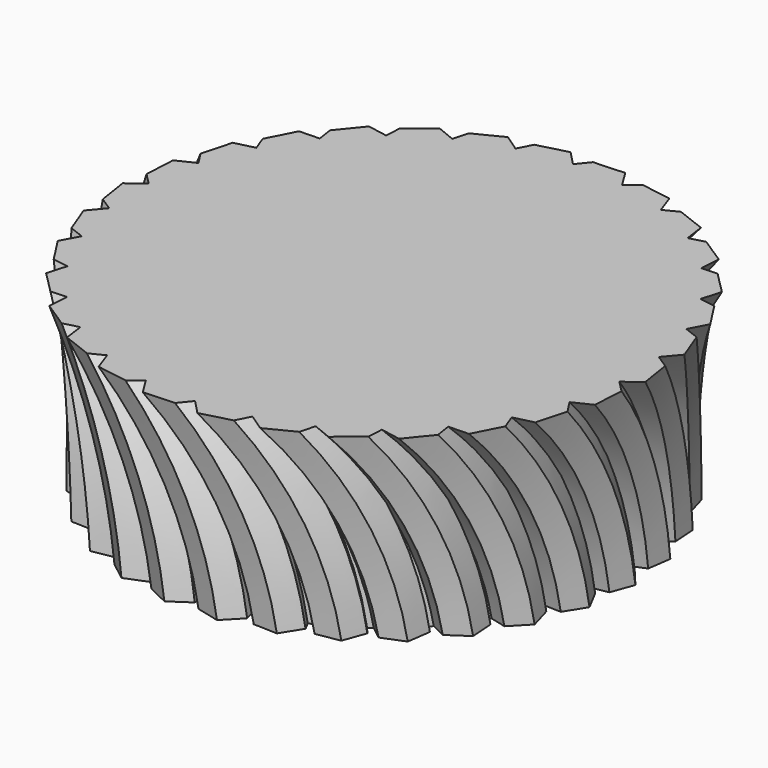
from build123d import *

# Parameters (mm, degrees)
F5_COUNT = 30
F6_R     = 30
F7_DEPTH = 25
F8_R     = 86.1433169454
F9_DEPTH = 25


with BuildPart() as f4:
    # F4: sweep along a path in F2
    with BuildLine(Plane.YZ.offset(-30)) as f4_path:
        ThreePointArc((13.1748821586, 26.7821643502), (4.4397694253, 14.4475808429), (0, 0))
    # F0 (on Top) → F4 (sweep)
    with BuildSketch(Plane.XY):
        Polygon((-32.0411247972, 2.43251781), (-33.1271846172, -0.5514070217), (-31.08605982, -2.9839248316), (-27.9588752028, -2.43251781), (-26.8728153828, 0.5514070217), (-28.91394018, 2.9839248316), align=None)
        Polygon((-17.6281463431, 1.8192284857), (-28.91394018, 2.9839248316), (-26.8728153828, 0.5514070217), (-27.9588752028, -2.43251781), (-17.6281463431, -1.5337090503), align=None)
    sweep(path=f4_path.line)

    # F5: F4 ×30 about axis
    f5_axis = Axis((0, 0, 15.9086212516), (0, 0, 1))


with BuildPart() as f4_1:
    add(f4.part)
    for i in range(1, F5_COUNT):
        add(f4.part.rotate(f5_axis, i * 360 / F5_COUNT))

    # F6 (on Top) → F7 (join)
    with BuildSketch(Plane.XY):
        Circle(F6_R)
    extrude(amount=F7_DEPTH)

    # F8 (on face) → F9 (cut)
    with BuildSketch(Plane.XY.offset(25)):
        Circle(F8_R)
        with BuildLine():
            Line((-17.6281463431, 9.5111030199), (-17.6281463431, 13.1997105208))
            add(Edge.make_bspline(
                [(-17.6281463436, 13.1997105151), (-17.03748869, 13.1417822064), (-16.4468217334, 13.0839139825), (-15.8561453818, 13.0261064694), (-15.2654595405, 12.9683603114)],
                knots=[0.771630404, 0.771630404, 0.771630404, 0.771630404, 0.771630404, 1, 1, 1, 1, 1], degree=4))
            Line((-15.2654595405, 12.9683603114), (-14.4985549182, 16.5763628885))
            add(Edge.make_bspline(
                [(-14.4985549199, 16.5763628831), (-13.9328485257, 16.3968958154), (-13.3671205396, 16.2174855854), (-12.8013707413, 16.0381327862), (-12.2355989041, 15.8588380282)],
                knots=[0.771630404, 0.771630404, 0.771630404, 0.771630404, 0.771630404, 1, 1, 1, 1, 1], degree=4))
            Line((-12.2355989041, 15.8588380282), (-10.7353070716, 19.2285486557))
            add(Edge.make_bspline(
                [(-10.7353070744, 19.2285486508), (-10.2192760237, 18.9353863962), (-9.7032120357, 18.642275248), (-9.1871147716, 18.3492157407), (-8.6709838828, 18.0562084241)],
                knots=[0.771630404, 0.771630404, 0.771630404, 0.771630404, 0.771630404, 1, 1, 1, 1, 1], degree=4))
            Line((-8.6709838828, 18.0562084241), (-6.5028747922, 21.0403545779))
            add(Edge.make_bspline(
                [(-6.502874796, 21.0403545736), (-6.0590721219, 20.6463097294), (-5.6152266046, 20.2523080268), (-5.1713378016, 19.858349918), (-4.7274052577, 19.4644358685)],
                knots=[0.771630404, 0.771630404, 0.771630404, 0.771630404, 0.771630404, 1, 1, 1, 1, 1], degree=4))
            Line((-4.7274052577, 19.4644358685), (-1.9862356802, 21.9325960422))
            add(Edge.make_bspline(
                [(-1.9862356848, 21.9325960388), (-1.6340576937, 21.4548902555), (-1.2818288261, 20.9772177634), (-0.929548555, 20.4995789129), (-0.5772163383, 20.0219740647)],
                knots=[0.771630404, 0.771630404, 0.771630404, 0.771630404, 0.771630404, 1, 1, 1, 1, 1], degree=4))
            Line((-0.5772163383, 20.0219740647), (2.617211462, 21.8662778151))
            add(Edge.make_bspline(
                [(2.6172114569, 21.8662778128), (2.8623728968, 21.3257891254), (3.1075910231, 20.7853224239), (3.352866424, 20.2448779415), (3.5981997049, 19.7044559182)],
                knots=[0.771630404, 0.771630404, 0.771630404, 0.771630404, 0.771630404, 1, 1, 1, 1, 1], degree=4))
            Line((3.5981997049, 19.7044559182), (7.1062739047, 20.8442983215))
            add(Edge.make_bspline(
                [(7.1062738991, 20.8442983203), (7.2337040565, 20.264648678), (7.3611942326, 19.6850087554), (7.4887450515, 19.1053786583), (7.6163571549, 18.5257584956)],
                knots=[0.771630404, 0.771630404, 0.771630404, 0.771630404, 0.771630404, 1, 1, 1, 1, 1], degree=4))
            Line((7.6163571549, 18.5257584956), (11.2847580779, 18.9113229693))
            add(Edge.make_bspline(
                [(11.2847580723, 18.9113229692), (11.2888876377, 18.3178458429), (11.2930779313, 17.7243657452), (11.2973295851, 17.13088265), (11.3016432499, 16.5373965303)],
                knots=[0.771630404, 0.771630404, 0.771630404, 0.771630404, 0.771630404, 1, 1, 1, 1, 1], degree=4))
            Line((11.3016432499, 16.5373965303), (14.9700441729, 16.1518320566))
            add(Edge.make_bspline(
                [(14.9700441674, 16.1518320578), (14.8506926591, 15.5704652456), (14.7313999341, 14.989082901), (14.6121666054, 14.4076848668), (14.4929933036, 13.8262709814)],
                knots=[0.771630404, 0.771630404, 0.771630404, 0.771630404, 0.771630404, 1, 1, 1, 1, 1], degree=4))
            Line((14.4929933036, 13.8262709814), (18.0010675033, 12.686428578))
            add(Edge.make_bspline(
                [(18.0010674981, 12.6864285803), (17.7634511498, 12.1425806017), (17.5258890708, 11.5987052084), (17.288381828, 11.0548021191), (17.0509300048, 10.5108710448)],
                knots=[0.771630404, 0.771630404, 0.771630404, 0.771630404, 0.771630404, 1, 1, 1, 1, 1], degree=4))
            Line((17.0509300048, 10.5108710448), (20.2453578051, 8.6665672944))
            add(Edge.make_bspline(
                [(20.2453578005, 8.6665672977), (19.8998615867, 8.184006919), (19.5544127565, 7.7014084414), (19.2090118059, 7.218771472), (18.8636592453, 6.7360956068)],
                knots=[0.771630404, 0.771630404, 0.771630404, 0.771630404, 0.771630404, 1, 1, 1, 1, 1], degree=4))
            Line((18.8636592453, 6.7360956068), (21.6048288228, 4.2679354331))
            add(Edge.make_bspline(
                [(21.604828819, 4.2679354373), (21.1665525822, 3.8677528627), (20.7283147722, 3.4675231701), (20.2901157927, 3.0672458721), (19.851956059, 2.6669204674)],
                knots=[0.771630404, 0.771630404, 0.771630404, 0.771630404, 0.771630404, 1, 1, 1, 1, 1], degree=4))
            Line((19.851956059, 2.6669204674), (22.0200651495, -0.3172256864))
            add(Edge.make_bspline(
                [(22.0200651467, -0.3172256815), (21.5081636614, -0.6175405533), (20.996289967, -0.9179095028), (20.4844443567, -1.2183330907), (19.9726271326, -1.5188118938)],
                knots=[0.771630404, 0.771630404, 0.771630404, 0.771630404, 0.771630404, 1, 1, 1, 1, 1], degree=4))
            Line((19.9726271326, -1.5188118938), (21.4729189652, -4.8885225212))
            add(Edge.make_bspline(
                [(21.4729189634, -4.8885225158), (20.909764781, -5.0758444838), (20.3466265388, -5.2632251258), (19.783504407, -5.4506650512), (19.2203985613, -5.6381648871)],
                knots=[0.771630404, 0.771630404, 0.771630404, 0.771630404, 0.771630404, 1, 1, 1, 1, 1], degree=4))
            Line((19.2203985613, -5.6381648871), (19.9873031836, -9.2461674641))
            add(Edge.make_bspline(
                [(19.9873031829, -9.2461674585), (19.3975088435, -9.3123096537), (18.8077178969, -9.378512555), (18.217930383, -9.4447767938), (17.6281463431, -9.5111030199)],
                knots=[0.771630404, 0.771630404, 0.771630404, 0.771630404, 0.771630404, 1, 1, 1, 1, 1], degree=4))
            Line((17.6281463431, -9.5111030199), (17.6281463431, -13.1997105208))
            add(Edge.make_bspline(
                [(17.6281463436, -13.1997105151), (17.03748869, -13.1417822064), (16.4468217334, -13.0839139825), (15.8561453818, -13.0261064694), (15.2654595405, -12.9683603114)],
                knots=[0.771630404, 0.771630404, 0.771630404, 0.771630404, 0.771630404, 1, 1, 1, 1, 1], degree=4))
            Line((15.2654595405, -12.9683603114), (14.4985549182, -16.5763628885))
            add(Edge.make_bspline(
                [(14.4985549199, -16.5763628831), (13.9328485257, -16.3968958154), (13.3671205396, -16.2174855854), (12.8013707413, -16.0381327862), (12.2355989041, -15.8588380282)],
                knots=[0.771630404, 0.771630404, 0.771630404, 0.771630404, 0.771630404, 1, 1, 1, 1, 1], degree=4))
            Line((12.2355989041, -15.8588380282), (10.7353070716, -19.2285486557))
            add(Edge.make_bspline(
                [(10.7353070744, -19.2285486508), (10.2192760237, -18.9353863962), (9.7032120357, -18.642275248), (9.1871147716, -18.3492157407), (8.6709838828, -18.0562084241)],
                knots=[0.771630404, 0.771630404, 0.771630404, 0.771630404, 0.771630404, 1, 1, 1, 1, 1], degree=4))
            Line((8.6709838828, -18.0562084241), (6.5028747922, -21.0403545779))
            add(Edge.make_bspline(
                [(6.502874796, -21.0403545736), (6.0590721219, -20.6463097294), (5.6152266046, -20.2523080268), (5.1713378016, -19.858349918), (4.7274052577, -19.4644358685)],
                knots=[0.771630404, 0.771630404, 0.771630404, 0.771630404, 0.771630404, 1, 1, 1, 1, 1], degree=4))
            Line((4.7274052577, -19.4644358685), (1.9862356802, -21.9325960422))
            add(Edge.make_bspline(
                [(1.9862356848, -21.9325960388), (1.6340576937, -21.4548902555), (1.2818288261, -20.9772177634), (0.929548555, -20.4995789129), (0.5772163383, -20.0219740647)],
                knots=[0.771630404, 0.771630404, 0.771630404, 0.771630404, 0.771630404, 1, 1, 1, 1, 1], degree=4))
            Line((0.5772163383, -20.0219740647), (-2.617211462, -21.8662778151))
            add(Edge.make_bspline(
                [(-2.6172114569, -21.8662778128), (-2.8623728968, -21.3257891254), (-3.1075910231, -20.7853224239), (-3.352866424, -20.2448779415), (-3.5981997049, -19.7044559182)],
                knots=[0.771630404, 0.771630404, 0.771630404, 0.771630404, 0.771630404, 1, 1, 1, 1, 1], degree=4))
            Line((-3.5981997049, -19.7044559182), (-7.1062739047, -20.8442983215))
            add(Edge.make_bspline(
                [(-7.1062738991, -20.8442983203), (-7.2337040565, -20.264648678), (-7.3611942326, -19.6850087554), (-7.4887450515, -19.1053786583), (-7.6163571549, -18.5257584956)],
                knots=[0.771630404, 0.771630404, 0.771630404, 0.771630404, 0.771630404, 1, 1, 1, 1, 1], degree=4))
            Line((-7.6163571549, -18.5257584956), (-11.2847580779, -18.9113229693))
            add(Edge.make_bspline(
                [(-11.2847580723, -18.9113229692), (-11.2888876377, -18.3178458429), (-11.2930779313, -17.7243657452), (-11.2973295851, -17.13088265), (-11.3016432499, -16.5373965303)],
                knots=[0.771630404, 0.771630404, 0.771630404, 0.771630404, 0.771630404, 1, 1, 1, 1, 1], degree=4))
            Line((-11.3016432499, -16.5373965303), (-14.9700441729, -16.1518320566))
            add(Edge.make_bspline(
                [(-14.9700441674, -16.1518320578), (-14.8506926591, -15.5704652456), (-14.7313999341, -14.989082901), (-14.6121666054, -14.4076848668), (-14.4929933036, -13.8262709814)],
                knots=[0.771630404, 0.771630404, 0.771630404, 0.771630404, 0.771630404, 1, 1, 1, 1, 1], degree=4))
            Line((-14.4929933036, -13.8262709814), (-18.0010675033, -12.686428578))
            add(Edge.make_bspline(
                [(-18.0010674981, -12.6864285803), (-17.7634511498, -12.1425806017), (-17.5258890708, -11.5987052084), (-17.288381828, -11.0548021191), (-17.0509300048, -10.5108710448)],
                knots=[0.771630404, 0.771630404, 0.771630404, 0.771630404, 0.771630404, 1, 1, 1, 1, 1], degree=4))
            Line((-17.0509300048, -10.5108710448), (-20.2453578051, -8.6665672944))
            add(Edge.make_bspline(
                [(-20.2453578005, -8.6665672977), (-19.8998615867, -8.184006919), (-19.5544127565, -7.7014084414), (-19.2090118059, -7.218771472), (-18.8636592453, -6.7360956068)],
                knots=[0.771630404, 0.771630404, 0.771630404, 0.771630404, 0.771630404, 1, 1, 1, 1, 1], degree=4))
            Line((-18.8636592453, -6.7360956068), (-21.6048288228, -4.2679354331))
            add(Edge.make_bspline(
                [(-21.604828819, -4.2679354373), (-21.1665525822, -3.8677528627), (-20.7283147722, -3.4675231701), (-20.2901157927, -3.0672458721), (-19.851956059, -2.6669204674)],
                knots=[0.771630404, 0.771630404, 0.771630404, 0.771630404, 0.771630404, 1, 1, 1, 1, 1], degree=4))
            Line((-19.851956059, -2.6669204674), (-22.0200651495, 0.3172256864))
            add(Edge.make_bspline(
                [(-22.0200651467, 0.3172256815), (-21.5081636614, 0.6175405533), (-20.996289967, 0.9179095028), (-20.4844443567, 1.2183330907), (-19.9726271326, 1.5188118938)],
                knots=[0.771630404, 0.771630404, 0.771630404, 0.771630404, 0.771630404, 1, 1, 1, 1, 1], degree=4))
            Line((-19.9726271326, 1.5188118938), (-21.4729189652, 4.8885225212))
            add(Edge.make_bspline(
                [(-21.4729189634, 4.8885225158), (-20.909764781, 5.0758444838), (-20.3466265388, 5.2632251258), (-19.783504407, 5.4506650512), (-19.2203985613, 5.6381648871)],
                knots=[0.771630404, 0.771630404, 0.771630404, 0.771630404, 0.771630404, 1, 1, 1, 1, 1], degree=4))
            Line((-19.2203985613, 5.6381648871), (-19.9873031836, 9.2461674641))
            add(Edge.make_bspline(
                [(-19.9873031829, 9.2461674585), (-19.3975088435, 9.3123096537), (-18.8077178969, 9.378512555), (-18.217930383, 9.4447767938), (-17.6281463431, 9.5111030199)],
                knots=[0.771630404, 0.771630404, 0.771630404, 0.771630404, 0.771630404, 1, 1, 1, 1, 1], degree=4))
        make_face(mode=Mode.SUBTRACT)
    extrude(amount=F9_DEPTH, mode=Mode.SUBTRACT)


solid = f4_1.part
